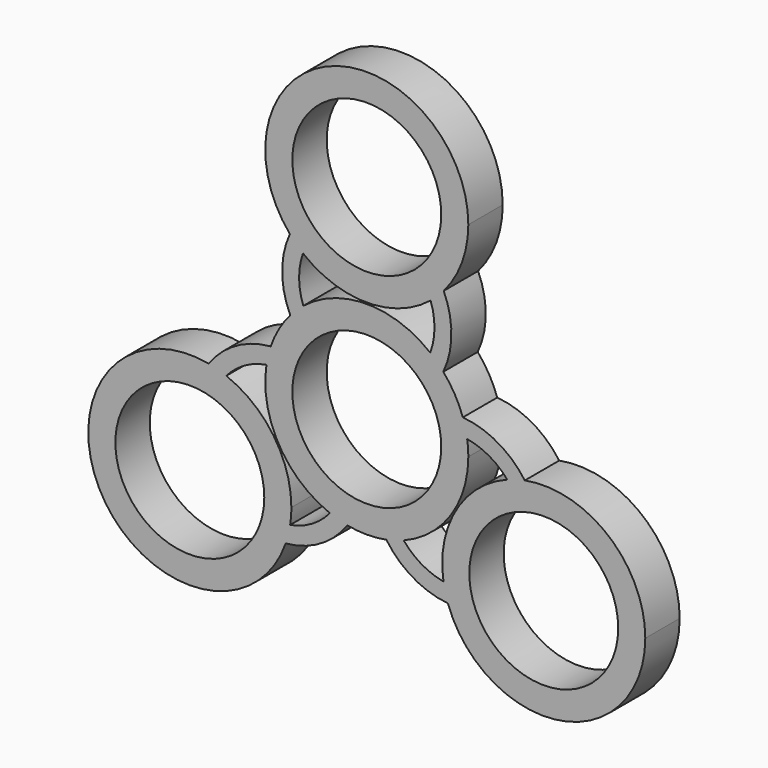
from build123d import *

# Parameters (mm, degrees)
F0_R     = 11
F1_DEPTH = 6.35


# Not quite as in the source:
# - a length typed as a fraction of an inch, garbled in the dataset ("3 / 203.2 mm" for 3/8 in), is restored


with BuildPart() as f1:
    # F0 (on Front) → F1 (new body)
    with BuildSketch(Plane.XZ):
        with BuildLine():
            ThreePointArc((5.4528368022, -13.9737815501), (12.3853250267, -8.4618983676), (15, 0))
            ThreePointArc((15, 0), (14.956955291, 1.1355564373), (14.8280682104, 2.2645955817))
            ThreePointArc((14.8280682104, 2.2645955817), (14.5670313108, 3.5779321946), (14.1899117897, 4.8627567696))
            ThreePointArc((14.1899117897, 4.8627567696), (12.9903810568, 7.5), (11.3062267898, 9.8574457025))
            ThreePointArc((11.3062267898, 9.8574457025), (10.382095829, 10.8264530756), (9.3752314082, 11.7091859684))
            ThreePointArc((9.3752314082, 11.7091859684), (0, 15), (-9.3752314082, 11.7091859684))
            ThreePointArc((-9.3752314082, 11.7091859684), (-10.382095829, 10.8264530756), (-11.3062267898, 9.8574457025))
            ThreePointArc((-11.3062267898, 9.8574457025), (-12.9903810568, 7.5), (-14.1899117897, 4.8627567696))
            ThreePointArc((-14.1899117897, 4.8627567696), (-14.5670313108, 3.5779321946), (-14.8280682104, 2.2645955817))
            ThreePointArc((-14.8280682104, 2.2645955817), (-12.9903810568, -7.5), (-5.4528368022, -13.9737815501))
            ThreePointArc((-5.4528368022, -13.9737815501), (-4.1849354819, -14.4043852702), (-2.883685, -14.7202024721))
            ThreePointArc((-2.883685, -14.7202024721), (0, -15), (2.883685, -14.7202024721))
            ThreePointArc((2.883685, -14.7202024721), (4.1849354819, -14.4043852702), (5.4528368022, -13.9737815501))
        make_face()
        Circle(F0_R, mode=Mode.SUBTRACT)
        with BuildLine():
            ThreePointArc((14.1899117897, 4.8627567696), (14.5670313108, 3.5779321946), (14.8280682104, 2.2645955817))
            ThreePointArc((14.8280682104, 2.2645955817), (18.0862095917, 1.1045798418), (20.7543499599, -1.0959084571))
            ThreePointArc((20.7543499599, -1.0959084571), (22.0334229862, -0.6684079546), (23.3457232771, -0.3575182103))
            ThreePointArc((23.3457232771, -0.3575182103), (19.3449005461, 3.2647619918), (14.1899117897, 4.8627567696))
        make_face()
        with BuildLine():
            ThreePointArc((11.326259544, -17.4258400757), (8.0865105924, -16.2154068855), (5.4528368022, -13.9737815501))
            ThreePointArc((5.4528368022, -13.9737815501), (4.1849354819, -14.4043852702), (2.883685, -14.7202024721))
            ThreePointArc((2.883685, -14.7202024722), (6.8450834508, -18.3855563025), (11.982481491, -20.0392303225))
            ThreePointArc((11.982481491, -20.0392303225), (11.5955697619, -18.7473000611), (11.326259544, -17.4258400757))
        make_face()
        with BuildLine():
            ThreePointArc((23.3457232771, -0.3575182103), (22.0334229862, -0.6684079546), (20.7543499599, -1.0959084571))
            ThreePointArc((20.7543499599, -1.0959084571), (13.153553406, -7.5942075998), (11.326259544, -17.4258400757))
            ThreePointArc((11.326259544, -17.4258400757), (11.5955697619, -18.7473000611), (11.982481491, -20.0392303225))
            ThreePointArc((11.982481491, -20.0392303225), (28.6517428111, -29.8830850855), (41.1439344628, -15.0942075998))
            ThreePointArc((41.1439344628, -15.0942075998), (35.7101989431, -3.5405681778), (23.3457232771, -0.3575182103))
        make_face()
        with Locations((26.1439344628, -15.0942075998)):
            Circle(F0_R, mode=Mode.SUBTRACT)
        with BuildLine():
            ThreePointArc((9.3752314082, 11.7091859684), (10.382095829, 10.8264530756), (11.3062267898, 9.8574457025))
            ThreePointArc((11.3062267898, 9.8574457025), (12.4998170953, 15.1207943107), (11.3632417861, 20.3967485329))
            ThreePointArc((11.3632417861, 20.3967485329), (10.4378532243, 19.4157080157), (9.4280904158, 18.5217485329))
            ThreePointArc((9.4280904158, 18.5217485329), (9.9996989994, 15.1108270437), (9.3752314082, 11.7091859684))
        make_face()
        with BuildLine():
            ThreePointArc((-11.982481491, -20.0392303225), (-6.8450834508, -18.3855563025), (-2.883685, -14.7202024722))
            ThreePointArc((-2.883685, -14.7202024721), (-4.1849354819, -14.4043852702), (-5.4528368022, -13.9737815501))
            ThreePointArc((-5.4528368022, -13.9737815501), (-8.0865105924, -16.2154068855), (-11.326259544, -17.4258400757))
            ThreePointArc((-11.326259544, -17.4258400757), (-11.5955697619, -18.7473000611), (-11.982481491, -20.0392303225))
        make_face()
        with BuildLine():
            ThreePointArc((9.4280904158, 18.5217485329), (10.4378532243, 19.4157080157), (11.3632417861, 20.3967485329))
            ThreePointArc((11.3632417861, 20.3967485329), (14.0614477703, 24.9658021941), (15, 30.1884151995))
            ThreePointArc((15, 30.1884151995), (-5.2226130054, 44.2498629698), (-11.3632417861, 20.3967485329))
            ThreePointArc((-11.3632417861, 20.3967485329), (-10.4378532243, 19.4157080157), (-9.4280904158, 18.5217485329))
            ThreePointArc((-9.4280904158, 18.5217485329), (0, 15.1884151995), (9.4280904158, 18.5217485329))
        make_face()
        with Locations((0, 30.1884151995)):
            Circle(F0_R, mode=Mode.SUBTRACT)
        with BuildLine():
            ThreePointArc((-23.3457232771, -0.3575182103), (-39.1343155195, -22.5942075998), (-11.982481491, -20.0392303225))
            ThreePointArc((-11.982481491, -20.0392303225), (-11.5955697619, -18.7473000611), (-11.326259544, -17.4258400757))
            ThreePointArc((-11.326259544, -17.4258400757), (-11.1895851994, -16.2635826934), (-11.1439344628, -15.0942075998))
            ThreePointArc((-11.1439344628, -15.0942075998), (-13.7777756504, -6.6043244305), (-20.7543499599, -1.0959084571))
            ThreePointArc((-20.7543499599, -1.0959084571), (-22.0334229862, -0.6684079546), (-23.3457232771, -0.3575182103))
        make_face()
        with Locations((-26.1439344628, -15.0942075998)):
            Circle(F0_R, mode=Mode.SUBTRACT)
        with BuildLine():
            ThreePointArc((-11.3062267898, 9.8574457025), (-10.382095829, 10.8264530756), (-9.3752314082, 11.7091859684))
            ThreePointArc((-9.3752314082, 11.7091859684), (-9.9996989994, 15.1108270437), (-9.4280904158, 18.5217485329))
            ThreePointArc((-9.4280904158, 18.5217485329), (-10.4378532243, 19.4157080157), (-11.3632417861, 20.3967485329))
            ThreePointArc((-11.3632417861, 20.3967485329), (-12.4998170953, 15.1207943107), (-11.3062267898, 9.8574457025))
        make_face()
        with BuildLine():
            ThreePointArc((-20.7543499599, -1.0959084571), (-18.0862095917, 1.1045798418), (-14.8280682104, 2.2645955817))
            ThreePointArc((-14.8280682104, 2.2645955817), (-14.5670313108, 3.5779321946), (-14.1899117897, 4.8627567696))
            ThreePointArc((-14.1899117897, 4.8627567696), (-19.3449005461, 3.2647619918), (-23.3457232771, -0.3575182103))
            ThreePointArc((-23.3457232771, -0.3575182103), (-22.0334229862, -0.6684079546), (-20.7543499599, -1.0959084571))
        make_face()
    extrude(amount=-F1_DEPTH)


solid = f1.part
